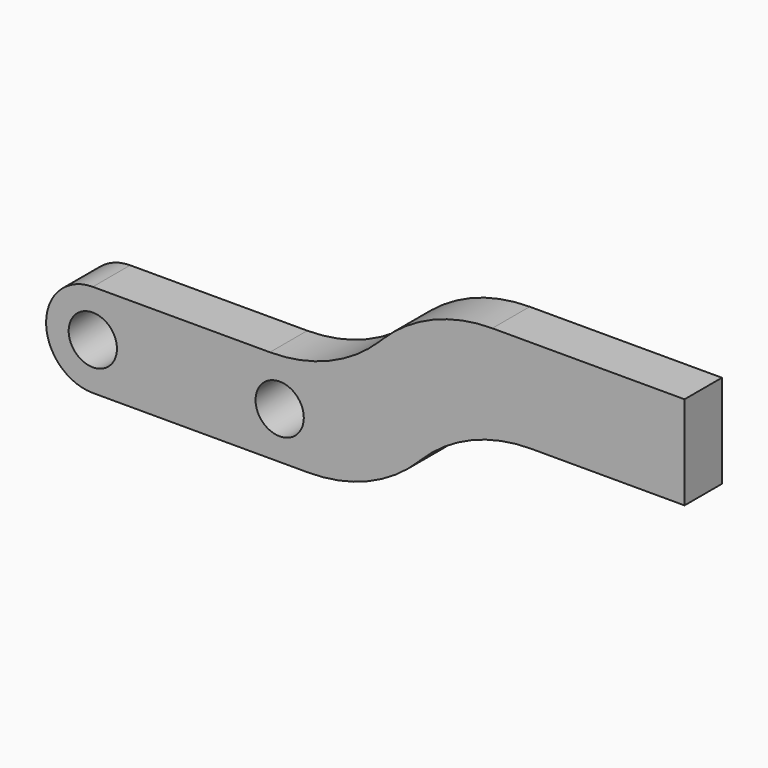
from build123d import *

# Parameters (mm, degrees)
F1_DEPTH = 7.5
F2_R     = 50
F3_R     = 14.99999
F4_R     = 7.75
F5_DEPTH = 15


# Not quite as in the source:
# - a fillet or chamfer is up to 0.001 mm smaller than in the source, because OpenCascade refuses the exact size


with BuildPart() as f1:
    # F0 (on Front) → F1 (new body, symmetric)
    with BuildSketch(Plane.XZ):
        Polygon((92.5735931288, 0), (0, 0), (0, -30), (105, -30), (135, 0), (205, 0), (205, 30), (122.5735931288, 30), align=None)
    extrude(amount=F1_DEPTH, both=True)

    # F2
    f2_edges = [f1.edges().sort_by_distance(p)[0] for p in [
        (92.573593, 0, 0),
        (122.573593, 0, 30),
        (105, 0, -30),
        (135, 0, 0),
    ]]
    fillet(f2_edges, radius=F2_R)

    # F3 (radius 15 in the source; OpenCascade refuses exactly that, so slightly less here)
    f3_edges = [f1.edges().sort_by_distance(p)[0] for p in [
        (0, 0, 0),
        (0, 0, -30),
    ]]
    fillet(f3_edges, radius=F3_R)

    # F4 (on face) → F5 (cut, through all)
    with BuildSketch(Plane.XZ.offset(7.5)):
        with Locations((15, -15)):
            Circle(F4_R)
        with Locations((75, -15)):
            Circle(F4_R)
    extrude(amount=-F5_DEPTH, mode=Mode.SUBTRACT)


solid = f1.part
